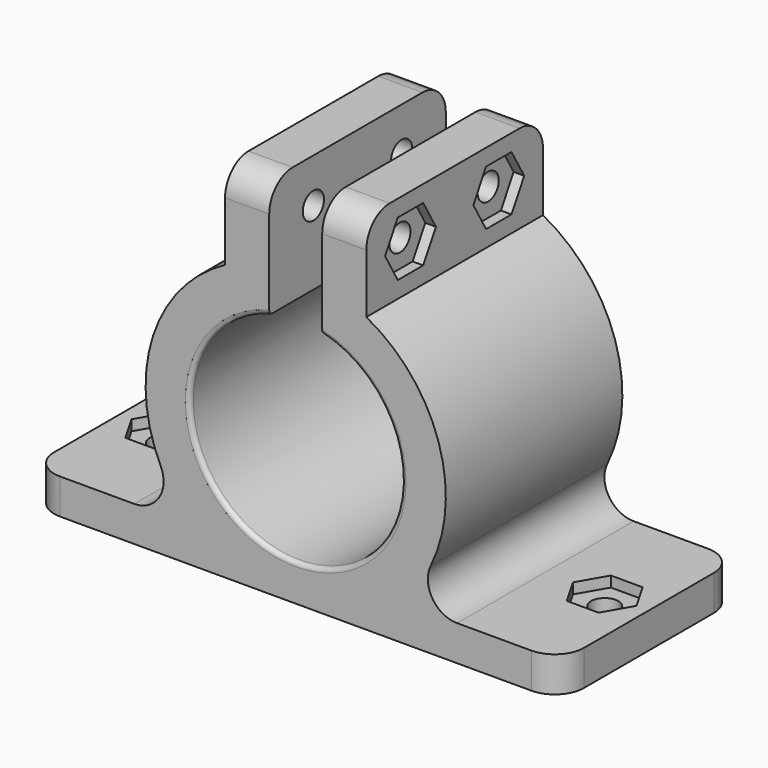
from build123d import *

# Parameters (mm, degrees)
F1_DEPTH  = 25
F2_R      = 1.55
F3_DEPTH  = 25
F4_R      = 1.5
F5_DEPTH  = 25
F6_R      = 3.3134143982
F9_DEPTH  = 1.2
F8_R      = 1.5
F10_DEPTH = 1.2
F12_DEPTH = 1.2
F13_R     = 0.5


# Not quite as in the source:
# - ends of sketch curves that miss each other by under 0.0002 mm in the source are joined


with BuildPart() as f1:
    # F0 (on Front) → F1 (new body)
    with BuildSketch(Plane.XZ):
        with BuildLine():
            Line((-30, -26.7712218283), (30, -26.771222222))
            Line((30, -26.771222222), (30, -22.771222222))
            Line((30, -22.771222222), (11.8647393899, -22.7712218283))
            ThreePointArc((11.8647393899, -22.7712218283), (16.8306466966, -8.2027211962), (8, 4.4036710302))
            Line((8, 4.4036710302), (8, 14.4036710302))
            Line((8, 14.4036710302), (3, 14.4036710302))
            Line((3, 14.4036710302), (3, 6.1368714524))
            Line((3, 6.1368714524), (3, 4.8868714524))
            Line((3, 4.8868714524), (3, 1.0226200218))
            ThreePointArc((3, 1.0226200218), (0, -22.5963300169), (-3, 1.0226200218))
            Line((-3, 1.0226200218), (-3, 4.8868714524))
            Line((-3, 4.8868714524), (-3, 14.4036710302))
            Line((-3, 14.4036710302), (-8, 14.4036710302))
            Line((-8, 14.4036710302), (-8, 4.4036710302))
            ThreePointArc((-8, 4.4036710302), (-16.8306466966, -8.2027211962), (-11.8647393899, -22.7712218283))
            Line((-11.8647393899, -22.7712218283), (-30, -22.7712218283))
            Line((-30, -22.7712218283), (-30, -26.7712218283))
        make_face()
    extrude(amount=F1_DEPTH)

    # F2 (on face) → F3 (cut)
    with BuildSketch(Plane.XY.offset(-22.7712218283)):
        with Locations((-25, -12.5)):
            Circle(F2_R)
        with Locations((25, -12.5)):
            Circle(F2_R)
    extrude(amount=-F3_DEPTH, mode=Mode.SUBTRACT)

    # F4 (on face) → F5 (cut)
    with BuildSketch(Plane.YZ.offset(8)):
        with Locations((-18.75, 9.4036710302)):
            Circle(F4_R)
        with Locations((-6.25, 9.4036710302)):
            Circle(F4_R)
    extrude(amount=-F5_DEPTH, mode=Mode.SUBTRACT)

    # F6
    f6_edges = [f1.edges().sort_by_distance(p)[0] for p in [
        (-5.5, -25, 14.403671),
        (5.5, -25, 14.403671),
        (-5.5, 0, 14.403671),
        (5.5, 0, 14.403671),
        (30, -25, -24.771222),
        (30, 0, -24.771222),
        (-30, 0, -24.771222),
        (-30, -25, -24.771222),
        (11.864739, -12.5, -22.771222),
        (-11.864739, -12.5, -22.771222),
    ]]
    fillet(f6_edges, radius=F6_R)

    # F7 (on face) → F9 (cut)
    with BuildSketch(Plane.YZ.offset(8)):
        Polygon((-20.55, 6.2859795766), (-16.95, 6.2859795766), (-15.15, 9.4036710302), (-16.95, 12.5213624838), (-20.55, 12.5213624838), (-22.35, 9.4036710302), align=None)
        Polygon((-4.45, 12.5213624838), (-8.05, 12.5213624838), (-9.85, 9.4036710302), (-8.05, 6.2859795766), (-4.45, 6.2859795766), (-2.65, 9.4036710302), align=None)
    extrude(amount=-F9_DEPTH, mode=Mode.SUBTRACT)

    # F8 (on face) → F10 (cut)
    with BuildSketch(Plane(origin=(-8, 0, 0), x_dir=(0, -1, 0), z_dir=(-1, 0, 0))):
        Polygon((4.45, 6.2859795766), (8.05, 6.2859795766), (9.85, 9.4036710302), (8.05, 12.5213624838), (4.45, 12.5213624838), (2.65, 9.4036710302), align=None)
        with Locations((6.25, 9.4036710302)):
            Circle(F8_R, mode=Mode.SUBTRACT)
        Polygon((20.55, 12.5213624838), (16.95, 12.5213624838), (15.15, 9.4036710302), (16.95, 6.2859795766), (20.55, 6.2859795766), (22.35, 9.4036710302), align=None)
        with Locations((18.75, 9.4036710302)):
            Circle(F8_R, mode=Mode.SUBTRACT)
    extrude(amount=-F10_DEPTH, mode=Mode.SUBTRACT)

    # F11 (on face) → F12 (cut)
    with BuildSketch(Plane.XY.offset(-22.7712218283)):
        Polygon((26.8, -9.3823085464), (23.2, -9.3823085464), (21.4, -12.5), (23.2, -15.6176914536), (26.8, -15.6176914536), (28.6, -12.5), align=None)
        Polygon((-23.2, -15.6176914536), (-21.4, -12.5), (-23.2, -9.3823085464), (-26.8, -9.3823085464), (-28.6, -12.5), (-26.8, -15.6176914536), align=None)
    extrude(amount=-F12_DEPTH, mode=Mode.SUBTRACT)

    # F13
    f13_edges = [f1.edges().sort_by_distance(p)[0] for p in [
        (0, 0, -22.59633),
        (0, -25, -22.59633),
    ]]
    fillet(f13_edges, radius=F13_R)


solid = f1.part
